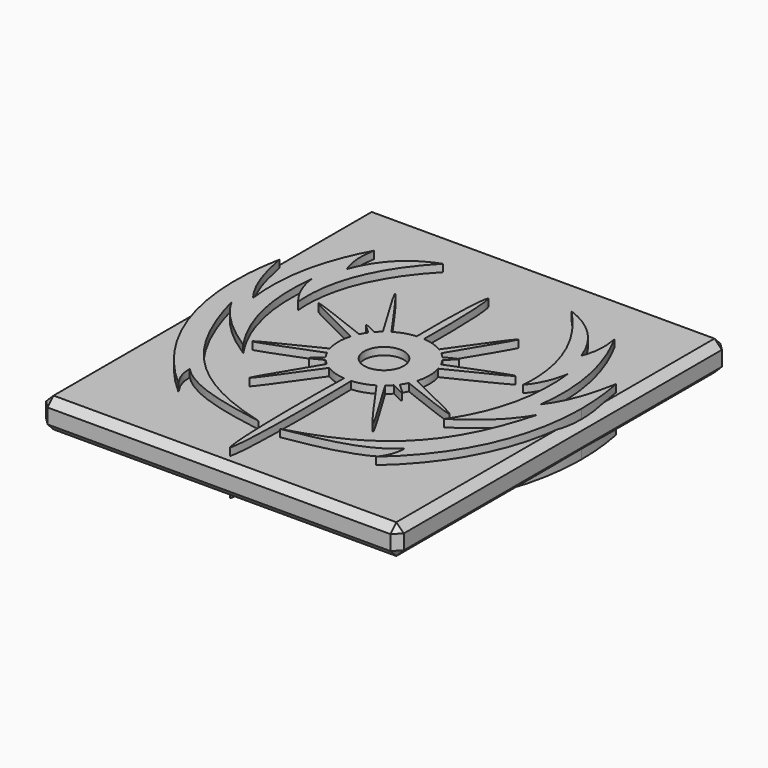
from build123d import *

# Parameters (mm, degrees)
F1_DEPTH     = 9.525
F0_R         = 8.4433652374
F2_DEPTH     = 6.35
F3_T1_DEPTH  = 4.0327916303
F3_T3_DEPTH  = 4.0327916303
F3_T5_DEPTH  = 4.0327916303
F3_T7_DEPTH  = 4.0327916303
F3_T9_DEPTH  = 4.0327916303
F3_T11_DEPTH = 4.0327916303
F3_T13_DEPTH = 4.0327916303
F3_T15_DEPTH = 4.0327916303
F3_T17_DEPTH = 168.7301869736
F3_T19_DEPTH = 29.0301869736
F3_T21_DEPTH = 192.1295813736


# Not quite as in the source:
# - a fillet or chamfer that OpenCascade refuses, or shapes differently, is made with other operations: its cross-section is extruded or revolved along the edge and cut away or added


with BuildPart() as f1:
    # F0 (on Top) → F1 (new body, symmetric)
    with BuildSketch(Plane.XY):
        with BuildLine():
            add(Edge.make_bspline(
                [(-29.2606507263, 77.812652531), (-42.8091961953, 63.8208179818), (-51.5423805175, 46.3544493376), (-49.7669426482, 26.4014893174)],
                knots=[0, 0, 0, 0, 55.3499386753, 55.3499386753, 55.3499386753, 55.3499386753], degree=3))
            add(Edge.make_bspline(
                [(-51.7986784398, 54.8546531534), (-48.0304780097, 65.5601248883), (-40.4704092019, 73.7719270438), (-29.2606507263, 77.812652531)],
                knots=[0, 0, 0, 0, 32.1719198779, 32.1719198779, 32.1719198779, 32.1719198779], degree=3))
            add(Edge.make_bspline(
                [(-53.0211725263, 70.9295149976), (-54.0685896293, 65.2563373521), (-53.9709406432, 60.4715305865), (-51.7986784398, 54.8546531534)],
                knots=[0, 0, 0, 0, 16.1212801943, 16.1212801943, 16.1212801943, 16.1212801943], degree=3))
            add(Edge.make_bspline(
                [(-63.1945773264, 19.0895324623), (-65.5408083551, 37.859361357), (-61.8847015844, 54.5059106867), (-53.0211725263, 70.9295149976)],
                knots=[0, 0, 0, 0, 52.8287985334, 52.8287985334, 52.8287985334, 52.8287985334], degree=3))
            add(Edge.make_bspline(
                [(-73.5923671773, 46.1759407263), (-71.7974136899, 36.5559011066), (-69.1904931891, 26.9102939647), (-63.1945773264, 19.0895324623)],
                knots=[0, 0, 0, 0, 29.0135752093, 29.0135752093, 29.0135752093, 29.0135752093], degree=3))
            add(Edge.make_bspline(
                [(-43.9423878337, -44.5992940976), (-71.1795652042, -20.7963531331), (-80.2357465407, 12.4160031447), (-73.5923671773, 46.1759407263)],
                knots=[0, 0, 0, 0, 95.4948403444, 95.4948403444, 95.4948403444, 95.4948403444], degree=3))
            add(Edge.make_bspline(
                [(-47.6710019998, -33.9658393011), (-47.8091001336, -37.1420657655), (-46.7043247304, -41.1468729767), (-43.9423878337, -44.5992940976)],
                knots=[0, 0, 0, 0, 11.2682263249, 11.2682263249, 11.2682263249, 11.2682263249], degree=3))
            add(Edge.make_bspline(
                [(-6.3993743878, -48.9143564549), (-24.6088343907, -45.8421644121), (-39.3851945322, -42.527841425), (-47.6710019998, -33.9658393011)],
                knots=[0, 0, 0, 0, 43.8953916811, 43.8953916811, 43.8953916811, 43.8953916811], degree=3))
            add(Edge.make_bspline(
                [(-6.3993743878, -48.9143564549), (-42.4233244741, -39.213518438), (-57.890164006, -21.260931832), (-67.0045570541, 12.5727854849)],
                knots=[0, 0, 0, 0, 86.3345631247, 86.3345631247, 86.3345631247, 86.3345631247], degree=3))
            add(Edge.make_bspline(
                [(-44.6424590731, -9.2521117545), (-52.9070365386, -3.8583881371), (-61.7805812079, 3.0142598604), (-67.0045570541, 12.5727854849)],
                knots=[0, 0, 0, 0, 31.2472329274, 31.2472329274, 31.2472329274, 31.2472329274], degree=3))
            add(Edge.make_bspline(
                [(-56.4955288244, 42.3137206278), (-58.561744892, 24.0671784128), (-55.5169024283, 6.7550672596), (-44.6424590731, -9.2521117545)],
                knots=[0, 0, 0, 0, 52.9105880879, 52.9105880879, 52.9105880879, 52.9105880879], degree=3))
            add(Edge.make_bspline(
                [(-49.7669426482, 26.4014893174), (-53.367226157, 30.5825783743), (-56.1044913938, 36.9695348902), (-56.4955288244, 42.3137206278)],
                knots=[0, 0, 0, 0, 17.2763704871, 17.2763704871, 17.2763704871, 17.2763704871], degree=3))
        make_face()
    extrude(amount=F1_DEPTH, both=True)


with BuildPart() as f1b:
    # F0 (on Top) → F1, piece 2 (new body, symmetric)
    with BuildSketch(Plane.XY):
        with BuildLine():
            add(Edge.make_bspline(
                [(2.7021450713, -48.9143564549), (38.7260951576, -39.213518438), (54.1929346895, -21.260931832), (63.3073277376, 12.5727854849)],
                knots=[0, 0, 0, 0, 86.3345631247, 86.3345631247, 86.3345631247, 86.3345631247], degree=3))
            add(Edge.make_bspline(
                [(2.7021450713, -48.9143564549), (20.9116050742, -45.8421644121), (35.6879652158, -42.527841425), (43.9737726833, -33.9658393011)],
                knots=[0, 0, 0, 0, 43.8953916811, 43.8953916811, 43.8953916811, 43.8953916811], degree=3))
            add(Edge.make_bspline(
                [(43.9737726833, -33.9658393011), (44.1118708172, -37.1420657655), (43.007095414, -41.1468729767), (40.2451585173, -44.5992940976)],
                knots=[0, 0, 0, 0, 11.2682263249, 11.2682263249, 11.2682263249, 11.2682263249], degree=3))
            add(Edge.make_bspline(
                [(40.2451585173, -44.5992940976), (61.8128001538, -25.7510377737), (71.9806008529, -1.0028935843), (71.9806001418, 25.2452133015)],
                knots=[0, 0, 0, 0, 75.6171781925, 75.6171781925, 75.6171781925, 75.6171781925], degree=3))
            add(Edge.make_bspline(
                [(71.9806001418, 25.2452133015), (71.9805999548, 32.1451137379), (71.2779858771, 39.1486643719), (69.8951378608, 46.1759407263)],
                knots=[75.6171781925, 75.6171781925, 75.6171781925, 75.6171781925, 95.4948403444, 95.4948403444, 95.4948403444, 95.4948403444], degree=3))
            add(Edge.make_bspline(
                [(69.8951378608, 46.1759407263), (68.1001843735, 36.5559011066), (65.4932638727, 26.9102939647), (59.4973480099, 19.0895324623)],
                knots=[0, 0, 0, 0, 29.0135752093, 29.0135752093, 29.0135752093, 29.0135752093], degree=3))
            add(Edge.make_bspline(
                [(59.4973480099, 19.0895324623), (61.8435790386, 37.859361357), (58.187472268, 54.5059106867), (49.3239432098, 70.9295149976)],
                knots=[0, 0, 0, 0, 52.8287985334, 52.8287985334, 52.8287985334, 52.8287985334], degree=3))
            add(Edge.make_bspline(
                [(49.3239432098, 70.9295149976), (50.3713603129, 65.2563373521), (50.2737113267, 60.4715305865), (48.1014491233, 54.8546531534)],
                knots=[0, 0, 0, 0, 16.1212801943, 16.1212801943, 16.1212801943, 16.1212801943], degree=3))
            add(Edge.make_bspline(
                [(48.1014491233, 54.8546531534), (44.3332486932, 65.5601248883), (36.7731798855, 73.7719270438), (25.5634214099, 77.812652531)],
                knots=[0, 0, 0, 0, 32.1719198779, 32.1719198779, 32.1719198779, 32.1719198779], degree=3))
            add(Edge.make_bspline(
                [(25.5634214099, 77.812652531), (39.1119668789, 63.8208179818), (47.845151201, 46.3544493376), (46.0697133317, 26.4014893174)],
                knots=[0, 0, 0, 0, 55.3499386753, 55.3499386753, 55.3499386753, 55.3499386753], degree=3))
            add(Edge.make_bspline(
                [(46.0697133317, 26.4014893174), (49.6699968406, 30.5825783743), (52.4072620774, 36.9695348902), (52.798299508, 42.3137206278)],
                knots=[0, 0, 0, 0, 17.2763704871, 17.2763704871, 17.2763704871, 17.2763704871], degree=3))
            add(Edge.make_bspline(
                [(52.798299508, 42.3137206278), (54.8645155756, 24.0671784128), (51.8196731118, 6.7550672596), (40.9452297566, -9.2521117545)],
                knots=[0, 0, 0, 0, 52.9105880879, 52.9105880879, 52.9105880879, 52.9105880879], degree=3))
            add(Edge.make_bspline(
                [(40.9452297566, -9.2521117545), (49.2098072222, -3.8583881371), (58.0833518915, 3.0142598604), (63.3073277376, 12.5727854849)],
                knots=[0, 0, 0, 0, 31.2472329274, 31.2472329274, 31.2472329274, 31.2472329274], degree=3))
        make_face()
    extrude(amount=F1_DEPTH, both=True)


with BuildPart() as f1c:
    # F0 (on Top) → F1, piece 3 (new body, symmetric)
    with BuildSketch(Plane.XY):
        with BuildLine():
            ThreePointArc((16.7647761301, 6.6270157784), (17.3829151441, 9.3993824194), (17.5904384374, 12.2322337595))
            ThreePointArc((17.5904384374, 12.2322337595), (17.3829151441, 15.0650850997), (16.7647761301, 17.8374517406))
            ThreePointArc((16.7647761301, 17.8374517406), (16.2439404764, 19.3411179164), (15.6018604147, 20.7971450249))
            ThreePointArc((15.6018604147, 20.7971450249), (14.823002052, 22.2289322907), (13.9269351063, 23.590438498))
            ThreePointArc((13.9269351063, 23.590438498), (13.3259447038, 24.3817001439), (12.6853074979, 25.1412186931))
            ThreePointArc((12.6853074979, 25.1412186931), (11.6743587021, 26.1966878037), (10.5869682939, 27.1732197342))
            ThreePointArc((10.5869682939, 27.1732197342), (9.4509407415, 28.0498452424), (8.2533425014, 28.8402814112))
            ThreePointArc((8.2533425014, 28.8402814112), (4.1355367031, 30.7272795216), (-0.3071828123, 31.6100760832))
            ThreePointArc((-0.3071828123, 31.6100760832), (-1.8486146582, 31.6712868552), (-3.3900465042, 31.6100760832))
            ThreePointArc((-3.3900465042, 31.6100760832), (-7.8327660196, 30.7272795216), (-11.9505718179, 28.8402814112))
            ThreePointArc((-11.9505718179, 28.8402814112), (-13.148170058, 28.0498452424), (-14.2841976104, 27.1732197342))
            ThreePointArc((-14.2841976104, 27.1732197342), (-15.3715880185, 26.1966878037), (-16.3825368144, 25.1412186931))
            ThreePointArc((-16.3825368144, 25.1412186931), (-17.0231740202, 24.3817001439), (-17.6241644228, 23.590438498))
            ThreePointArc((-17.6241644228, 23.590438498), (-18.5202313685, 22.2289322907), (-19.2990897312, 20.7971450249))
            ThreePointArc((-19.2990897312, 20.7971450249), (-19.9411697929, 19.3411179164), (-20.4620054466, 17.8374517406))
            ThreePointArc((-20.4620054466, 17.8374517406), (-21.2876677539, 12.2322337595), (-20.4620054466, 6.6270157784))
            ThreePointArc((-20.4620054466, 6.6270157784), (-19.9411697929, 5.1233496027), (-19.2990897312, 3.6673224942))
            ThreePointArc((-19.2990897312, 3.6673224942), (-18.5202313685, 2.2355352284), (-17.6241644228, 0.8740290211))
            ThreePointArc((-17.6241644228, 0.8740290211), (-17.0231740202, 0.0827673752), (-16.3825368144, -0.676751174))
            ThreePointArc((-16.3825368144, -0.676751174), (-15.3715880185, -1.7322202846), (-14.2841976104, -2.7087522152))
            ThreePointArc((-14.2841976104, -2.7087522152), (-13.148170058, -3.5853777234), (-11.9505718179, -4.3758138921))
            ThreePointArc((-11.9505718179, -4.3758138921), (-7.8327660196, -6.2628120025), (-3.3900465042, -7.1456085641))
            ThreePointArc((-3.3900465042, -7.1456085641), (-1.8486146582, -7.2068193361), (-0.3071828123, -7.1456085641))
            ThreePointArc((-0.3071828123, -7.1456085641), (4.1355367031, -6.2628120025), (8.2533425014, -4.3758138921))
            ThreePointArc((8.2533425014, -4.3758138921), (9.4509407415, -3.5853777234), (10.5869682939, -2.7087522152))
            ThreePointArc((10.5869682939, -2.7087522152), (11.6743587021, -1.7322202846), (12.6853074979, -0.676751174))
            ThreePointArc((12.6853074979, -0.676751174), (13.3259447038, 0.0827673752), (13.9269351063, 0.8740290211))
            ThreePointArc((13.9269351063, 0.8740290211), (14.823002052, 2.2355352284), (15.6018604147, 3.6673224942))
            ThreePointArc((15.6018604147, 3.6673224942), (16.2439404764, 5.1233496027), (16.7647761301, 6.6270157784))
        make_face()
        with Locations((-1.8486146582, 12.2322337595)):
            Circle(F0_R, mode=Mode.SUBTRACT)
        with BuildLine():
            ThreePointArc((15.6018604147, 20.7971450249), (16.2439404764, 19.3411179164), (16.7647761301, 17.8374517406))
            add(Edge.make_bspline(
                [(16.7647761301, 17.8374517406), (28.572768942, 23.590438498), (52.1313798822, 35.0730440151), (27.7775403506, 25.5557679072), (15.6018604147, 20.7971450249)],
                knots=[0, 0, 0, 0, 0.5005860011, 1, 1, 1, 1], degree=3))
        make_face()
        with BuildLine():
            ThreePointArc((12.6853074979, 25.1412186931), (13.3259447038, 24.3817001439), (13.9269351063, 23.590438498))
            add(Edge.make_bspline(
                [(13.9269351063, 23.590438498), (16.0163260258, 25.3993869323), (20.2181217092, 29.0356227168), (15.2133320796, 26.4508442319), (12.6853074979, 25.1412186931)],
                knots=[0, 0, 0, 0, 0.4964630431, 1, 1, 1, 1], degree=3))
        make_face()
        with BuildLine():
            ThreePointArc((8.2533425014, 28.8402814112), (9.4509407415, 28.0498452424), (10.5869682939, 27.1732197342))
            add(Edge.make_bspline(
                [(10.5869682939, 27.1732197342), (17.6984584279, 38.9329383393), (31.9048501643, 62.4226973375), (16.1342770449, 40.0314400531), (8.2533425014, 28.8402814112)],
                knots=[0, 0, 0, 0, 0.5005430897, 1, 1, 1, 1], degree=3))
        make_face()
        with BuildLine():
            ThreePointArc((-3.3900465042, 31.6100760832), (-1.8486146582, 31.6712868552), (-0.3071828123, 31.6100760832))
            add(Edge.make_bspline(
                [(-0.3071828123, 31.6100760832), (-0.0784399797, 44.8785130448), (-0.42681479, 65.5487815964), (-1.8486146582, 67.8008375222)],
                knots=[0, 0, 0, 0, 36.22357279, 36.22357279, 36.22357279, 36.22357279], degree=3))
            add(Edge.make_bspline(
                [(-3.3900465042, 31.6100760832), (-3.6187893367, 44.8785130448), (-3.2704145264, 65.5487815964), (-1.8486146582, 67.8008375222)],
                knots=[0, 0, 0, 0, 36.22357279, 36.22357279, 36.22357279, 36.22357279], degree=3))
        make_face()
        with BuildLine():
            ThreePointArc((-14.2841976104, 27.1732197342), (-13.148170058, 28.0498452424), (-11.9505718179, 28.8402814112))
            add(Edge.make_bspline(
                [(-14.2841976104, 27.1732197342), (-21.3956877443, 38.9329383393), (-35.6020794808, 62.4226973375), (-19.8315063614, 40.0314400531), (-11.9505718179, 28.8402814112)],
                knots=[0, 0, 0, 0, 0.5005430897, 1, 1, 1, 1], degree=3))
        make_face()
        with BuildLine():
            ThreePointArc((-17.6241644228, 23.590438498), (-17.0231740202, 24.3817001439), (-16.3825368144, 25.1412186931))
            add(Edge.make_bspline(
                [(-17.6241644228, 23.590438498), (-19.7135553423, 25.3993869323), (-23.9153510257, 29.0356227168), (-18.9105613961, 26.4508442319), (-16.3825368144, 25.1412186931)],
                knots=[0, 0, 0, 0, 0.4964630431, 1, 1, 1, 1], degree=3))
        make_face()
        with BuildLine():
            ThreePointArc((-20.4620054466, 17.8374517406), (-19.9411697929, 19.3411179164), (-19.2990897312, 20.7971450249))
            add(Edge.make_bspline(
                [(-20.4620054466, 17.8374517406), (-32.2699982584, 23.590438498), (-55.8286091986, 35.0730440151), (-31.474769667, 25.5557679072), (-19.2990897312, 20.7971450249)],
                knots=[0, 0, 0, 0, 0.5005860011, 1, 1, 1, 1], degree=3))
        make_face()
        with BuildLine():
            add(Edge.make_bspline(
                [(-20.4620054466, 6.6270157784), (-32.2699982584, 0.8740290211), (-55.8286091986, -10.6085764961), (-31.474769667, -1.0913003881), (-19.2990897312, 3.6673224942)],
                knots=[0, 0, 0, 0, 0.5005860011, 1, 1, 1, 1], degree=3))
            ThreePointArc((-19.2990897312, 3.6673224942), (-19.9411697929, 5.1233496027), (-20.4620054466, 6.6270157784))
        make_face()
        with BuildLine():
            add(Edge.make_bspline(
                [(-17.6241644228, 0.8740290211), (-19.7135553423, -0.9349194132), (-23.9153510257, -4.5711551977), (-18.9105613961, -1.9863767128), (-16.3825368144, -0.676751174)],
                knots=[0, 0, 0, 0, 0.4964630431, 1, 1, 1, 1], degree=3))
            ThreePointArc((-16.3825368144, -0.676751174), (-17.0231740202, 0.0827673752), (-17.6241644228, 0.8740290211))
        make_face()
        with BuildLine():
            add(Edge.make_bspline(
                [(-14.2841976104, -2.7087522152), (-21.3956877443, -14.4684708203), (-35.6020794808, -37.9582298185), (-19.8315063614, -15.5669725341), (-11.9505718179, -4.3758138921)],
                knots=[0, 0, 0, 0, 0.5005430897, 1, 1, 1, 1], degree=3))
            ThreePointArc((-11.9505718179, -4.3758138921), (-13.148170058, -3.5853777234), (-14.2841976104, -2.7087522152))
        make_face()
        with BuildLine():
            add(Edge.make_bspline(
                [(-1.8486146582, -69.8211616454), (-0.0047923681, -65.5245353599), (0.227460728, -27.7838741159), (-0.3071828123, -7.1456085641)],
                knots=[0, 0, 0, 0, 62.6945050717, 62.6945050717, 62.6945050717, 62.6945050717], degree=3))
            ThreePointArc((-0.3071828123, -7.1456085641), (-1.8486146582, -7.2068193361), (-3.3900465042, -7.1456085641))
            add(Edge.make_bspline(
                [(-1.8486146582, -69.8211616454), (-3.6924369484, -65.5245353599), (-3.9246900445, -27.7838741159), (-3.3900465042, -7.1456085641)],
                knots=[0, 0, 0, 0, 62.6945050717, 62.6945050717, 62.6945050717, 62.6945050717], degree=3))
        make_face()
        with BuildLine():
            add(Edge.make_bspline(
                [(10.5869682939, -2.7087522152), (17.6984584279, -14.4684708203), (31.9048501643, -37.9582298185), (16.1342770449, -15.5669725341), (8.2533425014, -4.3758138921)],
                knots=[0, 0, 0, 0, 0.5005430897, 1, 1, 1, 1], degree=3))
            ThreePointArc((10.5869682939, -2.7087522152), (9.4509407415, -3.5853777234), (8.2533425014, -4.3758138921))
        make_face()
        with BuildLine():
            add(Edge.make_bspline(
                [(13.9269351063, 0.8740290211), (16.0163260258, -0.9349194132), (20.2181217092, -4.5711551977), (15.2133320796, -1.9863767128), (12.6853074979, -0.676751174)],
                knots=[0, 0, 0, 0, 0.4964630431, 1, 1, 1, 1], degree=3))
            ThreePointArc((13.9269351063, 0.8740290211), (13.3259447038, 0.0827673752), (12.6853074979, -0.676751174))
        make_face()
        with BuildLine():
            add(Edge.make_bspline(
                [(16.7647761301, 6.6270157784), (28.572768942, 0.8740290211), (52.1313798822, -10.6085764961), (27.7775403506, -1.0913003881), (15.6018604147, 3.6673224942)],
                knots=[0, 0, 0, 0, 0.5005860011, 1, 1, 1, 1], degree=3))
            ThreePointArc((16.7647761301, 6.6270157784), (16.2439404764, 5.1233496027), (15.6018604147, 3.6673224942))
        make_face()
    extrude(amount=F1_DEPTH, both=True)


with BuildPart() as f2:
    # F0 (on Top) → F2 (new body, symmetric)
    with BuildSketch(Plane.XY):
        Polygon((74.3513853418, -75.6674634405), (74.3513853418, 12.2322337595), (74.3513853418, 100.1319309595), (-78.0486146582, 100.1319309595), (-78.0486146582, -75.6674634405), align=None)
        with BuildLine():
            ThreePointArc((16.7647761301, 17.8374517406), (17.3829151441, 15.0650850997), (17.5904384374, 12.2322337595))
            ThreePointArc((17.5904384374, 12.2322337595), (17.3829151441, 9.3993824194), (16.7647761301, 6.6270157784))
            add(Edge.make_bspline(
                [(16.7647761301, 6.6270157784), (28.572768942, 0.8740290211), (52.1313798822, -10.6085764961), (27.7775403506, -1.0913003881), (15.6018604147, 3.6673224942)],
                knots=[0, 0, 0, 0, 0.5005860011, 1, 1, 1, 1], degree=3))
            ThreePointArc((15.6018604147, 3.6673224942), (14.823002052, 2.2355352284), (13.9269351063, 0.8740290211))
            add(Edge.make_bspline(
                [(13.9269351063, 0.8740290211), (16.0163260258, -0.9349194132), (20.2181217092, -4.5711551977), (15.2133320796, -1.9863767128), (12.6853074979, -0.676751174)],
                knots=[0, 0, 0, 0, 0.4964630431, 1, 1, 1, 1], degree=3))
            ThreePointArc((12.6853074979, -0.676751174), (11.6743587021, -1.7322202846), (10.5869682939, -2.7087522152))
            add(Edge.make_bspline(
                [(10.5869682939, -2.7087522152), (17.6984584279, -14.4684708203), (31.9048501643, -37.9582298185), (16.1342770449, -15.5669725341), (8.2533425014, -4.3758138921)],
                knots=[0, 0, 0, 0, 0.5005430897, 1, 1, 1, 1], degree=3))
            ThreePointArc((8.2533425014, -4.3758138921), (4.1355367031, -6.2628120025), (-0.3071828123, -7.1456085641))
            add(Edge.make_bspline(
                [(-1.8486146582, -69.8211616454), (-0.0047923681, -65.5245353599), (0.227460728, -27.7838741159), (-0.3071828123, -7.1456085641)],
                knots=[0, 0, 0, 0, 62.6945050717, 62.6945050717, 62.6945050717, 62.6945050717], degree=3))
            add(Edge.make_bspline(
                [(-1.8486146582, -69.8211616454), (-3.6924369484, -65.5245353599), (-3.9246900445, -27.7838741159), (-3.3900465042, -7.1456085641)],
                knots=[0, 0, 0, 0, 62.6945050717, 62.6945050717, 62.6945050717, 62.6945050717], degree=3))
            ThreePointArc((-3.3900465042, -7.1456085641), (-7.8327660196, -6.2628120025), (-11.9505718179, -4.3758138921))
            add(Edge.make_bspline(
                [(-14.2841976104, -2.7087522152), (-21.3956877443, -14.4684708203), (-35.6020794808, -37.9582298185), (-19.8315063614, -15.5669725341), (-11.9505718179, -4.3758138921)],
                knots=[0, 0, 0, 0, 0.5005430897, 1, 1, 1, 1], degree=3))
            ThreePointArc((-14.2841976104, -2.7087522152), (-15.3715880185, -1.7322202846), (-16.3825368144, -0.676751174))
            add(Edge.make_bspline(
                [(-17.6241644228, 0.8740290211), (-19.7135553423, -0.9349194132), (-23.9153510257, -4.5711551977), (-18.9105613961, -1.9863767128), (-16.3825368144, -0.676751174)],
                knots=[0, 0, 0, 0, 0.4964630431, 1, 1, 1, 1], degree=3))
            ThreePointArc((-17.6241644228, 0.8740290211), (-18.5202313685, 2.2355352284), (-19.2990897312, 3.6673224942))
            add(Edge.make_bspline(
                [(-20.4620054466, 6.6270157784), (-32.2699982584, 0.8740290211), (-55.8286091986, -10.6085764961), (-31.474769667, -1.0913003881), (-19.2990897312, 3.6673224942)],
                knots=[0, 0, 0, 0, 0.5005860011, 1, 1, 1, 1], degree=3))
            ThreePointArc((-20.4620054466, 6.6270157784), (-21.2876677539, 12.2322337595), (-20.4620054466, 17.8374517406))
            add(Edge.make_bspline(
                [(-20.4620054466, 17.8374517406), (-32.2699982584, 23.590438498), (-55.8286091986, 35.0730440151), (-31.474769667, 25.5557679072), (-19.2990897312, 20.7971450249)],
                knots=[0, 0, 0, 0, 0.5005860011, 1, 1, 1, 1], degree=3))
            ThreePointArc((-19.2990897312, 20.7971450249), (-18.5202313685, 22.2289322907), (-17.6241644228, 23.590438498))
            add(Edge.make_bspline(
                [(-17.6241644228, 23.590438498), (-19.7135553423, 25.3993869323), (-23.9153510257, 29.0356227168), (-18.9105613961, 26.4508442319), (-16.3825368144, 25.1412186931)],
                knots=[0, 0, 0, 0, 0.4964630431, 1, 1, 1, 1], degree=3))
            ThreePointArc((-16.3825368144, 25.1412186931), (-15.3715880185, 26.1966878037), (-14.2841976104, 27.1732197342))
            add(Edge.make_bspline(
                [(-14.2841976104, 27.1732197342), (-21.3956877443, 38.9329383393), (-35.6020794808, 62.4226973375), (-19.8315063614, 40.0314400531), (-11.9505718179, 28.8402814112)],
                knots=[0, 0, 0, 0, 0.5005430897, 1, 1, 1, 1], degree=3))
            ThreePointArc((-11.9505718179, 28.8402814112), (-7.8327660196, 30.7272795216), (-3.3900465042, 31.6100760832))
            add(Edge.make_bspline(
                [(-3.3900465042, 31.6100760832), (-3.6187893367, 44.8785130448), (-3.2704145264, 65.5487815964), (-1.8486146582, 67.8008375222)],
                knots=[0, 0, 0, 0, 36.22357279, 36.22357279, 36.22357279, 36.22357279], degree=3))
            add(Edge.make_bspline(
                [(-0.3071828123, 31.6100760832), (-0.0784399797, 44.8785130448), (-0.42681479, 65.5487815964), (-1.8486146582, 67.8008375222)],
                knots=[0, 0, 0, 0, 36.22357279, 36.22357279, 36.22357279, 36.22357279], degree=3))
            ThreePointArc((-0.3071828123, 31.6100760832), (4.1355367031, 30.7272795216), (8.2533425014, 28.8402814112))
            add(Edge.make_bspline(
                [(10.5869682939, 27.1732197342), (17.6984584279, 38.9329383393), (31.9048501643, 62.4226973375), (16.1342770449, 40.0314400531), (8.2533425014, 28.8402814112)],
                knots=[0, 0, 0, 0, 0.5005430897, 1, 1, 1, 1], degree=3))
            ThreePointArc((10.5869682939, 27.1732197342), (11.6743587021, 26.1966878037), (12.6853074979, 25.1412186931))
            add(Edge.make_bspline(
                [(13.9269351063, 23.590438498), (16.0163260258, 25.3993869323), (20.2181217092, 29.0356227168), (15.2133320796, 26.4508442319), (12.6853074979, 25.1412186931)],
                knots=[0, 0, 0, 0, 0.4964630431, 1, 1, 1, 1], degree=3))
            ThreePointArc((13.9269351063, 23.590438498), (14.823002052, 22.2289322907), (15.6018604147, 20.7971450249))
            add(Edge.make_bspline(
                [(16.7647761301, 17.8374517406), (28.572768942, 23.590438498), (52.1313798822, 35.0730440151), (27.7775403506, 25.5557679072), (15.6018604147, 20.7971450249)],
                knots=[0, 0, 0, 0, 0.5005860011, 1, 1, 1, 1], degree=3))
        make_face(mode=Mode.SUBTRACT)
        with BuildLine():
            add(Edge.make_bspline(
                [(-51.7986784398, 54.8546531534), (-48.0304780097, 65.5601248883), (-40.4704092019, 73.7719270438), (-29.2606507263, 77.812652531)],
                knots=[0, 0, 0, 0, 32.1719198779, 32.1719198779, 32.1719198779, 32.1719198779], degree=3))
            add(Edge.make_bspline(
                [(-29.2606507263, 77.812652531), (-42.8091961953, 63.8208179818), (-51.5423805175, 46.3544493376), (-49.7669426482, 26.4014893174)],
                knots=[0, 0, 0, 0, 55.3499386753, 55.3499386753, 55.3499386753, 55.3499386753], degree=3))
            add(Edge.make_bspline(
                [(-49.7669426482, 26.4014893174), (-53.367226157, 30.5825783743), (-56.1044913938, 36.9695348902), (-56.4955288244, 42.3137206278)],
                knots=[0, 0, 0, 0, 17.2763704871, 17.2763704871, 17.2763704871, 17.2763704871], degree=3))
            add(Edge.make_bspline(
                [(-56.4955288244, 42.3137206278), (-58.561744892, 24.0671784128), (-55.5169024283, 6.7550672596), (-44.6424590731, -9.2521117545)],
                knots=[0, 0, 0, 0, 52.9105880879, 52.9105880879, 52.9105880879, 52.9105880879], degree=3))
            add(Edge.make_bspline(
                [(-44.6424590731, -9.2521117545), (-52.9070365386, -3.8583881371), (-61.7805812079, 3.0142598604), (-67.0045570541, 12.5727854849)],
                knots=[0, 0, 0, 0, 31.2472329274, 31.2472329274, 31.2472329274, 31.2472329274], degree=3))
            add(Edge.make_bspline(
                [(-6.3993743878, -48.9143564549), (-42.4233244741, -39.213518438), (-57.890164006, -21.260931832), (-67.0045570541, 12.5727854849)],
                knots=[0, 0, 0, 0, 86.3345631247, 86.3345631247, 86.3345631247, 86.3345631247], degree=3))
            add(Edge.make_bspline(
                [(-6.3993743878, -48.9143564549), (-24.6088343907, -45.8421644121), (-39.3851945322, -42.527841425), (-47.6710019998, -33.9658393011)],
                knots=[0, 0, 0, 0, 43.8953916811, 43.8953916811, 43.8953916811, 43.8953916811], degree=3))
            add(Edge.make_bspline(
                [(-47.6710019998, -33.9658393011), (-47.8091001336, -37.1420657655), (-46.7043247304, -41.1468729767), (-43.9423878337, -44.5992940976)],
                knots=[0, 0, 0, 0, 11.2682263249, 11.2682263249, 11.2682263249, 11.2682263249], degree=3))
            add(Edge.make_bspline(
                [(-43.9423878337, -44.5992940976), (-71.1795652042, -20.7963531331), (-80.2357465407, 12.4160031447), (-73.5923671773, 46.1759407263)],
                knots=[0, 0, 0, 0, 95.4948403444, 95.4948403444, 95.4948403444, 95.4948403444], degree=3))
            add(Edge.make_bspline(
                [(-73.5923671773, 46.1759407263), (-71.7974136899, 36.5559011066), (-69.1904931891, 26.9102939647), (-63.1945773264, 19.0895324623)],
                knots=[0, 0, 0, 0, 29.0135752093, 29.0135752093, 29.0135752093, 29.0135752093], degree=3))
            add(Edge.make_bspline(
                [(-63.1945773264, 19.0895324623), (-65.5408083551, 37.859361357), (-61.8847015844, 54.5059106867), (-53.0211725263, 70.9295149976)],
                knots=[0, 0, 0, 0, 52.8287985334, 52.8287985334, 52.8287985334, 52.8287985334], degree=3))
            add(Edge.make_bspline(
                [(-53.0211725263, 70.9295149976), (-54.0685896293, 65.2563373521), (-53.9709406432, 60.4715305865), (-51.7986784398, 54.8546531534)],
                knots=[0, 0, 0, 0, 16.1212801943, 16.1212801943, 16.1212801943, 16.1212801943], degree=3))
        make_face(mode=Mode.SUBTRACT)
        with BuildLine():
            add(Edge.make_bspline(
                [(2.7021450713, -48.9143564549), (20.9116050742, -45.8421644121), (35.6879652158, -42.527841425), (43.9737726833, -33.9658393011)],
                knots=[0, 0, 0, 0, 43.8953916811, 43.8953916811, 43.8953916811, 43.8953916811], degree=3))
            add(Edge.make_bspline(
                [(2.7021450713, -48.9143564549), (38.7260951576, -39.213518438), (54.1929346895, -21.260931832), (63.3073277376, 12.5727854849)],
                knots=[0, 0, 0, 0, 86.3345631247, 86.3345631247, 86.3345631247, 86.3345631247], degree=3))
            add(Edge.make_bspline(
                [(40.9452297566, -9.2521117545), (49.2098072222, -3.8583881371), (58.0833518915, 3.0142598604), (63.3073277376, 12.5727854849)],
                knots=[0, 0, 0, 0, 31.2472329274, 31.2472329274, 31.2472329274, 31.2472329274], degree=3))
            add(Edge.make_bspline(
                [(52.798299508, 42.3137206278), (54.8645155756, 24.0671784128), (51.8196731118, 6.7550672596), (40.9452297566, -9.2521117545)],
                knots=[0, 0, 0, 0, 52.9105880879, 52.9105880879, 52.9105880879, 52.9105880879], degree=3))
            add(Edge.make_bspline(
                [(46.0697133317, 26.4014893174), (49.6699968406, 30.5825783743), (52.4072620774, 36.9695348902), (52.798299508, 42.3137206278)],
                knots=[0, 0, 0, 0, 17.2763704871, 17.2763704871, 17.2763704871, 17.2763704871], degree=3))
            add(Edge.make_bspline(
                [(25.5634214099, 77.812652531), (39.1119668789, 63.8208179818), (47.845151201, 46.3544493376), (46.0697133317, 26.4014893174)],
                knots=[0, 0, 0, 0, 55.3499386753, 55.3499386753, 55.3499386753, 55.3499386753], degree=3))
            add(Edge.make_bspline(
                [(48.1014491233, 54.8546531534), (44.3332486932, 65.5601248883), (36.7731798855, 73.7719270438), (25.5634214099, 77.812652531)],
                knots=[0, 0, 0, 0, 32.1719198779, 32.1719198779, 32.1719198779, 32.1719198779], degree=3))
            add(Edge.make_bspline(
                [(49.3239432098, 70.9295149976), (50.3713603129, 65.2563373521), (50.2737113267, 60.4715305865), (48.1014491233, 54.8546531534)],
                knots=[0, 0, 0, 0, 16.1212801943, 16.1212801943, 16.1212801943, 16.1212801943], degree=3))
            add(Edge.make_bspline(
                [(59.4973480099, 19.0895324623), (61.8435790386, 37.859361357), (58.187472268, 54.5059106867), (49.3239432098, 70.9295149976)],
                knots=[0, 0, 0, 0, 52.8287985334, 52.8287985334, 52.8287985334, 52.8287985334], degree=3))
            add(Edge.make_bspline(
                [(69.8951378608, 46.1759407263), (68.1001843735, 36.5559011066), (65.4932638727, 26.9102939647), (59.4973480099, 19.0895324623)],
                knots=[0, 0, 0, 0, 29.0135752093, 29.0135752093, 29.0135752093, 29.0135752093], degree=3))
            add(Edge.make_bspline(
                [(71.9806001418, 25.2452133015), (71.9805999548, 32.1451137379), (71.2779858771, 39.1486643719), (69.8951378608, 46.1759407263)],
                knots=[75.6171781925, 75.6171781925, 75.6171781925, 75.6171781925, 95.4948403444, 95.4948403444, 95.4948403444, 95.4948403444], degree=3))
            add(Edge.make_bspline(
                [(40.2451585173, -44.5992940976), (61.8128001538, -25.7510377737), (71.9806008529, -1.0028935843), (71.9806001418, 25.2452133015)],
                knots=[0, 0, 0, 0, 75.6171781925, 75.6171781925, 75.6171781925, 75.6171781925], degree=3))
            add(Edge.make_bspline(
                [(43.9737726833, -33.9658393011), (44.1118708172, -37.1420657655), (43.007095414, -41.1468729767), (40.2451585173, -44.5992940976)],
                knots=[0, 0, 0, 0, 11.2682263249, 11.2682263249, 11.2682263249, 11.2682263249], degree=3))
        make_face(mode=Mode.SUBTRACT)
    extrude(amount=F2_DEPTH, both=True)

    # F3: chamfer of 3.175 on 12 edges, made by hand

    # F3_s2 → F3_t1 (cut)
    with BuildSketch(Plane(origin=(-51.2386926996, -51.2386926996, -51.2386926996), x_dir=(0.7071067812, -0.7071067812, 0), z_dir=(-0.5773502692, -0.5773502692, -0.5773502692))):
        Polygon((0.5613358572, 58.8657611339), (-3.9287922034, 58.8657611339), (-1.6837281731, 54.9771961673), align=None)
    extrude(amount=F3_T1_DEPTH, mode=Mode.SUBTRACT)

    # F3_s4 → F3_t3 (cut)
    with BuildSketch(Plane(origin=(50.0062829274, -50.0062829274, -50.0062829274), x_dir=(0.7071067812, 0.7071067812, 0), z_dir=(0.5773502692, -0.5773502692, -0.5773502692))):
        Polygon((1.3144562821, 57.356373586), (-3.1756717784, 57.356373586), (-0.9306077482, 53.4678086194), align=None)
    extrude(amount=F3_T3_DEPTH, mode=Mode.SUBTRACT)

    # F3_s6 → F3_t5 (cut)
    with BuildSketch(Plane(origin=(50.0062829274, -50.0062829274, 50.0062829274), x_dir=(0.7071067812, 0.7071067812, 0), z_dir=(0.5773502692, -0.5773502692, 0.5773502692))):
        Polygon((1.3144562821, -57.356373586), (-3.1756717784, -57.356373586), (-0.9306077482, -53.4678086194), align=None)
    extrude(amount=F3_T5_DEPTH, mode=Mode.SUBTRACT)

    # F3_s8 → F3_t7 (cut)
    with BuildSketch(Plane(origin=(-51.2386926996, -51.2386926996, 51.2386926996), x_dir=(0.7071067812, -0.7071067812, 0), z_dir=(-0.5773502692, -0.5773502692, 0.5773502692))):
        Polygon((0.5613358572, -58.8657611339), (-3.9287922034, -58.8657611339), (-1.6837281731, -54.9771961673), align=None)
    extrude(amount=F3_T7_DEPTH, mode=Mode.SUBTRACT)

    # F3_s10 → F3_t9 (cut)
    with BuildSketch(Plane(origin=(-59.3935152059, 59.3935152059, -59.3935152059), x_dir=(-0.7071067812, -0.7071067812, 0), z_dir=(-0.5773502692, 0.5773502692, -0.5773502692))):
        Polygon((-13.3701986775, 68.8533381757), (-17.860326738, 68.8533381757), (-15.6152627077, 64.964773209), align=None)
    extrude(amount=F3_T9_DEPTH, mode=Mode.SUBTRACT)

    # F3_s12 → F3_t11 (cut)
    with BuildSketch(Plane(origin=(-59.3935152059, 59.3935152059, 59.3935152059), x_dir=(-0.7071067812, -0.7071067812, 0), z_dir=(-0.5773502692, 0.5773502692, 0.5773502692))):
        Polygon((-13.3701986775, -68.8533381757), (-15.6152627077, -64.964773209), (-17.860326738, -68.8533381757), align=None)
    extrude(amount=F3_T11_DEPTH, mode=Mode.SUBTRACT)

    # F3_s14 → F3_t13 (cut)
    with BuildSketch(Plane(origin=(58.1611054338, 58.1611054338, -58.1611054338), x_dir=(-0.7071067812, 0.7071067812, 0), z_dir=(0.5773502692, 0.5773502692, -0.5773502692))):
        Polygon((15.9845345987, 67.3439506278), (20.4746626593, 67.3439506278), (18.229598629, 63.4553856611), align=None)
    extrude(amount=F3_T13_DEPTH, mode=Mode.SUBTRACT)

    # F3_s16 → F3_t15 (cut)
    with BuildSketch(Plane(origin=(58.1611054338, 58.1611054338, 58.1611054338), x_dir=(-0.7071067812, 0.7071067812, 0), z_dir=(0.5773502692, 0.5773502692, 0.5773502692))):
        Polygon((15.9845345987, -67.3439506278), (18.229598629, -63.4553856611), (20.4746626593, -67.3439506278), align=None)
    extrude(amount=F3_T15_DEPTH, mode=Mode.SUBTRACT)

    # F3_s18 → F3_t17 (cut)
    with BuildSketch(Plane.YZ.offset(-86.213708145)):
        Polygon((-75.6674634405, -3.175), (-72.4924634405, -6.35), (-75.6674634405, -6.35), align=None)
        Polygon((-75.6674634405, 3.175), (-72.4924634405, 6.35), (-75.6674634405, 6.35), align=None)
        Polygon((100.1319309595, -3.175), (96.9569309595, -6.35), (100.1319309595, -6.35), align=None)
        Polygon((96.9569309595, 6.35), (100.1319309595, 3.175), (100.1319309595, 6.35), align=None)
    extrude(amount=F3_T17_DEPTH, mode=Mode.SUBTRACT)

    # F3_s20 → F3_t19 (cut)
    with BuildSketch(Plane.XY.offset(-14.5150934868)):
        Polygon((74.3513853418, -72.4924634405), (71.1763853418, -75.6674634405), (74.3513853418, -75.6674634405), align=None)
        Polygon((-74.8736146582, -75.6674634405), (-78.0486146582, -72.4924634405), (-78.0486146582, -75.6674634405), align=None)
        Polygon((-78.0486146582, 96.9569309595), (-74.8736146582, 100.1319309595), (-78.0486146582, 100.1319309595), align=None)
        Polygon((74.3513853418, 96.9569309595), (71.1763853418, 100.1319309595), (74.3513853418, 100.1319309595), align=None)
    extrude(amount=F3_T19_DEPTH, mode=Mode.SUBTRACT)

    # F3_s22 → F3_t21 (cut)
    with BuildSketch(Plane.XZ.offset(-108.2970244463)):
        Polygon((-78.0486146582, -3.175), (-74.8736146582, -6.35), (-78.0486146582, -6.35), align=None)
        Polygon((-78.0486146582, 3.175), (-74.8736146582, 6.35), (-78.0486146582, 6.35), align=None)
        Polygon((74.3513853418, -3.175), (71.1763853418, -6.35), (74.3513853418, -6.35), align=None)
        Polygon((74.3513853418, 3.175), (71.1763853418, 6.35), (74.3513853418, 6.35), align=None)
    extrude(amount=F3_T21_DEPTH, mode=Mode.SUBTRACT)


with BuildPart() as f2b:
    # F0 (on Top) → F2, piece 2 (new body, symmetric)
    with BuildSketch(Plane.XY):
        with Locations((-1.8486146582, 12.2322337595)):
            Circle(F0_R)
    extrude(amount=F2_DEPTH, both=True)


solid = Compound([f1.part, f1b.part, f1c.part, f2.part, f2b.part])
